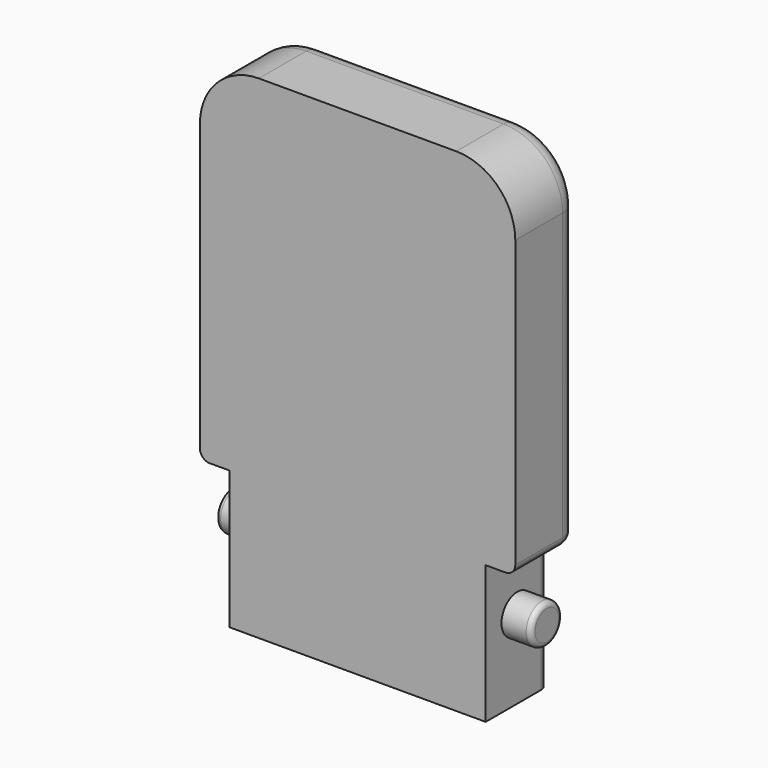
from build123d import *

# Parameters (mm, degrees)
F0_W        = 406.4
F0_H        = 635
F1_DEPTH    = 101.6
F2_W        = 129.6282266226
F2_H        = 559.1529050058
F2_W_2      = 230.7462543249
F2_H_2      = 486.9312153578
F3_DEPTH    = 127
F4_T1_DEPTH = 482.5995000003
F5_R        = 25.4
F6_R        = 25.4
F7_DEPTH    = 406.4
F8_R        = 6.35
F9_R        = 12.7
F10_DEPTH   = 25.4


# Not quite as in the source:
# - a fillet or chamfer that OpenCascade refuses, or shapes differently, is made with other operations: its cross-section is extruded or revolved along the edge and cut away or added
# - a feature names something its author has since deleted; it is built from what else it names


with BuildPart() as f1:
    # F0 (on Front) → F1 (new body)
    with BuildSketch(Plane.XZ):
        with Locations((-4.243819043, 96.6177646602)):
            Rectangle(F0_W, F0_H)
    extrude(amount=F1_DEPTH)

    # F2 (on face) → F3 (cut)
    with BuildSketch(Plane.XZ.offset(101.6)):
        with Locations((-234.1579323543, -322.6586878427)):
            Rectangle(F2_W, F2_H)
        with Locations((276.2293081194, -286.5478430187)):
            Rectangle(F2_W_2, F2_H_2)
    extrude(amount=-F3_DEPTH, mode=Mode.SUBTRACT)

    # F4: fillet of radius 76.2 on 2 edges, made by hand

    # F4_s2 → F4_t1 (cut)
    with BuildSketch(Plane.XZ.offset(-190.4997500002)):
        with BuildLine():
            ThreePointArc((198.956280957, 337.9178646602), (176.6378176834, 391.7994013866), (122.756280957, 414.1178646602))
            Line((122.756280957, 414.1178646602), (122.756280957, 415.6418646602))
            Line((122.756280957, 415.6418646602), (200.480180957, 415.6417646602))
            Line((200.480180957, 415.6417646602), (200.480280957, 337.9178646602))
            Line((200.480280957, 337.9178646602), (198.956280957, 337.9178646602))
        make_face()
        with BuildLine():
            ThreePointArc((-131.243919043, 414.1178646602), (-185.1254557695, 391.7994013866), (-207.443919043, 337.9178646602))
            Line((-207.443919043, 337.9178646602), (-208.967919043, 337.9178646602))
            Line((-208.967919043, 337.9178646602), (-208.967819043, 415.6417646602))
            Line((-208.967819043, 415.6417646602), (-131.243919043, 415.6418646602))
            Line((-131.243919043, 415.6418646602), (-131.243919043, 414.1178646602))
        make_face()
    extrude(amount=F4_T1_DEPTH, mode=Mode.SUBTRACT)

    # F5
    f5_edges = [f1.edges().sort_by_distance(p)[0] for p in [
        (198.956181, 0, 147.47954),
        (176.637818, 0, 391.799401),
        (-4.243819, 0, 414.117765),
        (-185.125456, 0, 391.799401),
        (-207.443819, 0, 147.47954),
    ]]
    fillet(f5_edges, radius=F5_R)

    # F6 (on face) → F7 (join)
    with BuildSketch(Plane.YZ.offset(198.956180957)):
        with Locations((-50.8, -119.2822353398)):
            Circle(F6_R)
    extrude(amount=-F7_DEPTH)

    # F8
    f8_edges = [f1.edges().sort_by_distance(p)[0] for p in [
        (-207.443819, -76.2, -119.282235),
        (198.956181, -76.2, -119.282235),
    ]]
    fillet(f8_edges, radius=F8_R)

    # F9
    f9_edges = [f1.edges().sort_by_distance(p)[0] for p in [
        (-169.343819, 0, -131.982235),
        (-175.693819, 0, -43.082235),
        (-200.004331, -7.439488, -43.082235),
        (-207.443819, -63.5, -43.082235),
        (160.856181, 0, -131.982235),
        (167.206181, 0, -43.082235),
        (191.516693, -7.439488, -43.082235),
        (198.956181, -63.5, -43.082235),
    ]]
    fillet(f9_edges, radius=F9_R)

    # F2 (on face) → F10 (cut)
    with BuildSketch(Plane.XZ.offset(101.6)):
        with Locations((-234.1579323543, -322.6586878427)):
            Rectangle(F2_W, F2_H)
        with Locations((276.2293081194, -286.5478430187)):
            Rectangle(F2_W_2, F2_H_2)
    extrude(amount=-F10_DEPTH, mode=Mode.SUBTRACT)


solid = f1.part
